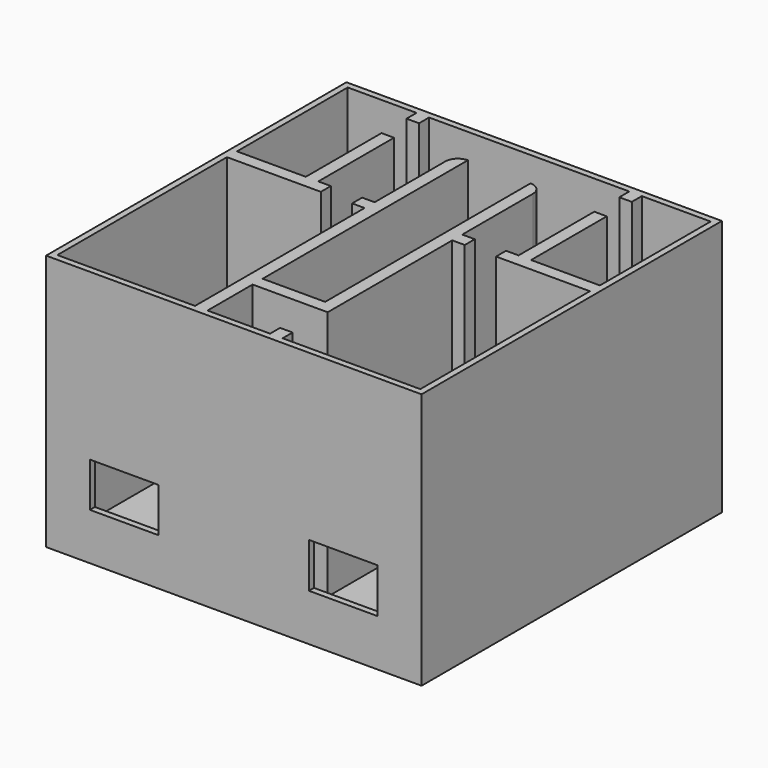
from build123d import *

# Parameters (mm, degrees)
F0_W      = 152.4
F0_H      = 152.4
F0_W_2    = 147.32
F0_H_2    = 147.32
F1_DEPTH  = 101.6
F2_W      = 152.4
F2_H      = 152.4
F3_DEPTH  = 2.54
F4_W      = 27.94
F4_H      = 18.1844604351
F4_H_2    = 17.9737907264
F5_DEPTH  = 25.4
F7_DEPTH  = 101.6
F8_W      = 25.4
F8_H      = 5.08
F9_DEPTH  = 101.6
F10_W     = 25.4
F10_H     = 5.08
F11_DEPTH = 101.6
F12_W     = 5.08
F12_H     = 5.08
F13_DEPTH = 101.6
F14_W     = 38.1
F14_H     = 5.08
F15_DEPTH = 101.6
F16_W     = 5.08
F16_H     = 38.4063468442
F16_H_2   = 5.08
F17_DEPTH = 101.6
F18_W     = 25.4
F18_H     = 104.14
F19_DEPTH = 25.4
F20_R     = 5.07999
F21_W     = 5.08
F21_H     = 5.08
F21_W_2   = 38.1
F21_H_2   = 22.86
F22_DEPTH = 101.6
F23_R     = 1.016
F24_DEPTH = 15.24


# Not quite as in the source:
# - a fillet or chamfer is up to 0.001 mm smaller than in the source, because OpenCascade refuses the exact size


with BuildPart() as f1:
    # F0 (on Top) → F1 (new body)
    with BuildSketch(Plane.XY):
        with Locations((-4.47035e-05, 5.21541e-05)):
            Rectangle(F0_W, F0_H)
        with Locations((-4.47035e-05, 5.21541e-05)):
            Rectangle(F0_W_2, F0_H_2, mode=Mode.SUBTRACT)
    extrude(amount=F1_DEPTH)

    # F2 (on face) → F3 (join)
    with BuildSketch(Plane(origin=(0, 0, 0), x_dir=(1, 0, 0), z_dir=(0, 0, -1))):
        with Locations((-4.47035e-05, -5.21541e-05)):
            Rectangle(F2_W, F2_H)
    extrude(amount=F3_DEPTH)

    # F4 (on face) → F5 (cut)
    with BuildSketch(Plane.XZ.offset(76.1999478459)):
        with Locations((44.4499552965, 25.6276302175)):
            Rectangle(F4_W, F4_H)
        with Locations((-44.4500447035, 25.5222953632)):
            Rectangle(F4_W, F4_H_2)
    extrude(amount=-F5_DEPTH, mode=Mode.SUBTRACT)

    # F6 (on face) → F7 (join)
    with BuildSketch(Plane.XY):
        Polygon((-17.7800447035, 58.4200521541), (-17.7800447035, -50.7999478459), (-12.7000447035, -50.7999478459), (-12.7000447035, 53.3400521541), (12.6999552965, 53.3400521541), (12.6999552965, -50.7999478459), (17.7799552965, -50.7999478459), (17.7799552965, 44.5264838636), (17.7799552965, 58.4200521541), align=None)
    extrude(amount=F7_DEPTH)

    # F8 (on face) → F9 (join)
    with BuildSketch(Plane.XY):
        with Locations((-4.47035e-05, -48.2599478459)):
            Rectangle(F8_W, F8_H)
    extrude(amount=F9_DEPTH)

    # F10 (on face) → F11 (cut)
    with BuildSketch(Plane.XY.offset(101.6)):
        with Locations((-4.47035e-05, 55.8800521541)):
            Rectangle(F10_W, F10_H)
    extrude(amount=-F11_DEPTH, mode=Mode.SUBTRACT)

    # F12 (on face) → F13 (join)
    with BuildSketch(Plane.XY):
        with Locations((-20.3200447035, 14.9337053099)):
            Rectangle(F12_W, F12_H)
    extrude(amount=F13_DEPTH)

    # F14 (on face) → F15 (join)
    with BuildSketch(Plane.XY):
        with Locations((-54.6100447035, 14.9337053099)):
            Rectangle(F14_W, F14_H)
    extrude(amount=F15_DEPTH)

    # F16 (on face) → F17 (join)
    with BuildSketch(Plane.XY):
        with Locations((-43.1800447035, 36.676878732)):
            Rectangle(F16_W, F16_H)
        with Locations((-43.1800447035, 71.1200521541)):
            Rectangle(F16_W, F16_H_2)
        with Locations((43.1799552965, 71.1200521541)):
            Rectangle(F16_W, F16_H_2)
        with Locations((43.1799552965, 36.676878732)):
            Rectangle(F16_W, F16_H)
    extrude(amount=F17_DEPTH)

    # F18 (on face) → F19 (cut)
    with BuildSketch(Plane.XY):
        with Locations((-4.47035e-05, 6.3500521541)):
            Rectangle(F18_W, F18_H)
    extrude(amount=-F19_DEPTH, mode=Mode.SUBTRACT)

    # F20 (radius 5.08 in the source; OpenCascade refuses exactly that, so slightly less here)
    f20_edges = [f1.edges().sort_by_distance(p)[0] for p in [
        (-17.780045, 58.420052, 50.8),
        (17.779955, 58.420052, 50.8),
    ]]
    fillet(f20_edges, radius=F20_R)

    # F21 (on face) → F22 (join)
    with BuildSketch(Plane.XY):
        with Locations((20.3199552965, 14.9337053099)):
            Rectangle(F21_W, F21_H)
        with Locations((54.6099552965, 14.9337053099)):
            Rectangle(F21_W_2, F21_H)
        with Locations((-15.2400447035, -62.2299478459)):
            Rectangle(F21_W, F21_H_2)
        with Locations((15.2399552965, -71.1199478459)):
            Rectangle(F21_W, F21_H)
    extrude(amount=F22_DEPTH)

    # F23 (on face) → F24 (cut)
    with BuildSketch(Plane(origin=(0, 0, -2.54), x_dir=(1, 0, 0), z_dir=(0, 0, -1))):
        with Locations((-74.9300447035, 74.9299478459)):
            Circle(F23_R)
        with Locations((74.9299552965, 74.9299478459)):
            Circle(F23_R)
        with Locations((-74.9300447035, -74.9300521541)):
            Circle(F23_R)
        with Locations((74.9299552965, -74.9300521541)):
            Circle(F23_R)
    extrude(amount=-F24_DEPTH, mode=Mode.SUBTRACT)


solid = f1.part
